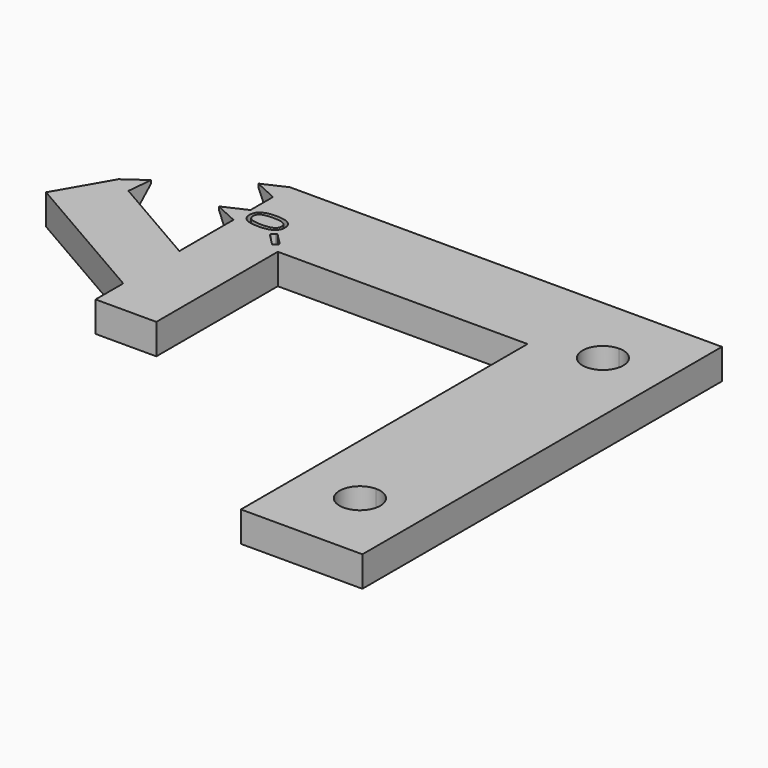
from build123d import *

# Parameters (mm, degrees)
F0_W         = 41.1068271101
F0_H         = 15
F1_DEPTH     = 5
F2_TEXT_SIZE = 7.8939358102
F3_DEPTH     = 2
F5_REACH     = 79.8703734186
F7_REACH     = 114.5656915951


# Not quite as in the source:
# - a feature names something its author has since deleted; it is built from what else it names
# - Text() gives the source's letters only with a copy of the font that has no kerning and outlines rounded to 1/6400 em; it was checked with that copy


with BuildPart() as f1:
    # F0 (on Top) → F1 (new body)
    with BuildSketch(Plane.XY):
        Polygon((11.2797634304, 17.1542509354), (11.2797634304, 11.4597389847), (21.2797634304, 11.4597389847), (21.2797634304, 22.9277536273), (16.2797634304, 14.2674995895), align=None)
        Polygon((-12.3231448688, 30.7813963956), (11.2797634304, 17.1542509354), (11.2797634304, 28.7012563192), (-4.2990511203, 37.6956890936), (-5.8110979945, 38.5686697635), (-7.3231448688, 39.4416504334), align=None)
        Polygon((11.2797634304, 28.7012563192), (11.2797634304, 17.1542509354), (16.2797634304, 14.2674995895), (21.2797634304, 22.9277536273), align=None)
        Polygon((11.2797634304, 28.7012563192), (21.2797634304, 22.9277536273), (21.2797634304, 36.4597389847), (21.2797634304, 51.4597389847), (11.2797634304, 51.4597389847), (11.2797634304, 49.7137776449), (11.2797634304, 47.9678163051), (11.2797634304, 43.3287542578), (11.2797634304, 41.5827929181), (11.2797634304, 39.8368315783), align=None)
        Polygon((7.4697634304, 41.5827929181), (11.2797634304, 39.8368315783), (11.2797634304, 41.5827929181), align=None)
        Polygon((7.4697634304, 41.5827929181), (11.2797634304, 41.5827929181), (11.2797634304, 43.3287542578), align=None)
        Polygon((11.2797634304, 47.9678163051), (11.2797634304, 49.7137776449), (7.4697634304, 49.7137776449), align=None)
        Polygon((11.2797634304, 49.7137776449), (11.2797634304, 51.4597389847), (7.4697634304, 49.7137776449), align=None)
        Polygon((-5.8110979945, 38.5686697635), (-4.2990511203, 37.6956890936), (-3.9060979945, 41.868226552), align=None)
        Polygon((-3.9060979945, 41.868226552), (-7.3231448688, 39.4416504334), (-5.8110979945, 38.5686697635), align=None)
        with Locations((41.8331769854, 43.9597389847)):
            Rectangle(F0_W, F0_H)
        with BuildLine():
            Line((62.3865905404, 51.4597389847), (62.3865905404, 36.4597389847))
            Line((62.3865905404, 36.4597389847), (62.3865905404, -22.5133558466))
            Line((62.3865905404, -22.5133558466), (72.3865905404, -22.5133558466))
            Line((72.3865905404, -22.5133558466), (72.3865905404, -13.879608431))
            ThreePointArc((72.3865905404, -13.879608431), (69.0337905404, -10.526808431), (72.3865905404, -7.174008431))
            Line((72.3865905404, -7.174008431), (72.3865905404, 36.120391569))
            ThreePointArc((72.3865905404, 36.120391569), (69.0337905404, 39.473191569), (72.3865905404, 42.825991569))
            Line((72.3865905404, 42.825991569), (72.3865905404, 51.4597389847))
            Line((72.3865905404, 51.4597389847), (62.3865905404, 51.4597389847))
        make_face()
        with BuildLine():
            Line((82.3865905404, 51.4597389847), (72.3865905404, 51.4597389847))
            Line((72.3865905404, 51.4597389847), (72.3865905404, 42.825991569))
            ThreePointArc((72.3865905404, 42.825991569), (74.7573781564, 41.843979185), (75.7393905404, 39.473191569))
            ThreePointArc((75.7393905404, 39.473191569), (74.7573781564, 37.1024039531), (72.3865905404, 36.120391569))
            Line((72.3865905404, 36.120391569), (72.3865905404, -7.174008431))
            ThreePointArc((72.3865905404, -7.174008431), (74.7573781564, -8.156020815), (75.7393905404, -10.526808431))
            ThreePointArc((75.7393905404, -10.526808431), (74.7573781564, -12.8975960469), (72.3865905404, -13.879608431))
            Line((72.3865905404, -13.879608431), (72.3865905404, -22.5133558466))
            Line((72.3865905404, -22.5133558466), (82.3865905404, -22.5133558466))
            Line((82.3865905404, -22.5133558466), (82.3865905404, 51.4597389847))
        make_face()
    extrude(amount=F1_DEPTH)

    # F2 (on face) → F3 (cut)
    with BuildSketch(Plane.XY.offset(5)):
        with BuildLine():
            Line((20.0423265633, 38.404282633), (18.2745596103, 40.1720495859))
            ThreePointArc((18.2745596103, 40.1720495859), (18.097782915, 40.2452728906), (17.9210062197, 40.1720495859))
            Line((17.9210062197, 40.1720495859), (17.5674528291, 39.8184961953))
            ThreePointArc((17.5674528291, 39.8184961953), (17.4942295244, 39.6417195), (17.5674528291, 39.4649428047))
            Line((17.5674528291, 39.4649428047), (19.3352197821, 37.6971758518))
            ThreePointArc((19.3352197821, 37.6971758518), (19.5119964774, 37.6239525471), (19.6887731727, 37.6971758518))
            Line((19.6887731727, 37.6971758518), (20.0423265633, 38.0507292424))
            ThreePointArc((20.0423265633, 38.0507292424), (20.115549868, 38.2275059377), (20.0423265633, 38.404282633))
        make_face()
        with Locations(Location((17.7442295244, 39.9952728906), (0, 0, 90))):
            Text('0', F2_TEXT_SIZE, font='Open Sans', text_align=(TextAlign.LEFT, TextAlign.BOTTOM))
    extrude(amount=-F3_DEPTH, mode=Mode.SUBTRACT)

    f5_end = f1.faces().sort_by_distance((3.4903561551, 33.1984727064, 2.5))[0]
    # F4 (on face) → F5 (cut, up to a face of the model that its end follows)
    with BuildSketch(Plane(origin=(0, 51.4597389847, 0), x_dir=(-1, 0, 0), z_dir=(0, 1, 0))):
        Polygon((-7.4697634304, 4.5), (-11.2797634304, 0), (-7.4697634304, 0), align=None)
    f5_long = extrude(amount=-F5_REACH, mode=Mode.PRIVATE)
    add(split(f5_long, bisect_by=f5_end, keep=Keep.TOP, mode=Mode.PRIVATE), mode=Mode.SUBTRACT)

    f7_end = f1.faces().sort_by_distance((11.2797634304, 34.2690439487, 2.5))[0]
    # F6 (on face) → F7 (cut, up to a face of the model that its end follows)
    with BuildSketch(Plane(origin=(-22.5710942729, 13.0314273543, 0), x_dir=(-0.5, -0.8660254038, 0), z_dir=(-0.8660254038, 0.5, 0))):
        Polygon((-34.3058988081, 0), (-30.4958988081, 0), (-34.3058988081, 4.5), align=None)
    f7_long = extrude(amount=-F7_REACH, mode=Mode.PRIVATE)
    add(split(f7_long, bisect_by=f7_end, keep=Keep.TOP, mode=Mode.PRIVATE), mode=Mode.SUBTRACT)


solid = f1.part
